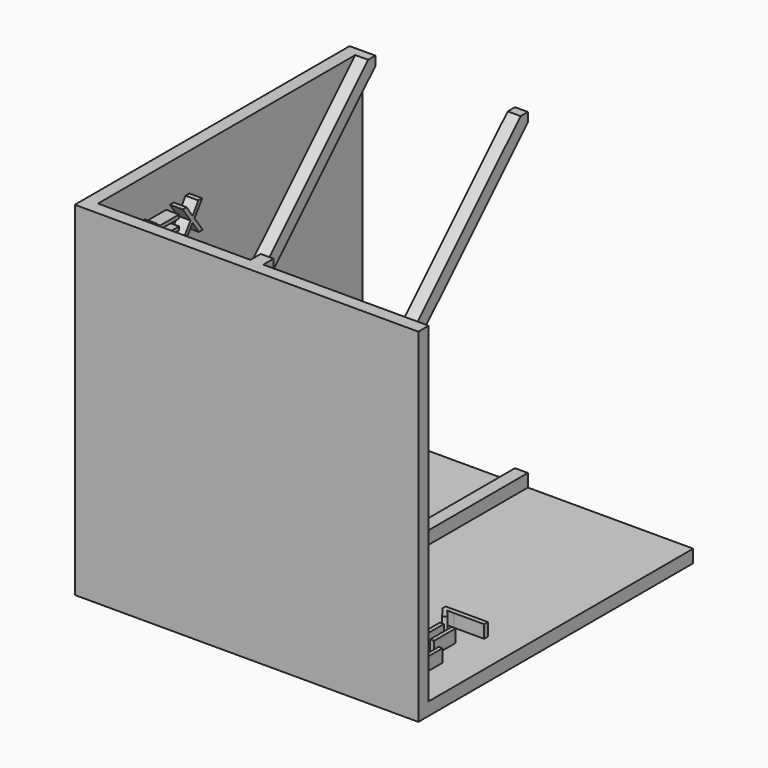
from build123d import *

# Parameters (mm, degrees)
F0_W          = 3.81
F0_H          = 203.2
F1_DEPTH      = 15.24
F0_W_2        = 97.79
F2_DEPTH      = 7.62
F3_W          = 97.79
F3_H          = 203.2
F4_DEPTH      = 7.62
F3_W_2        = 3.81
F5_DEPTH      = 15.24
F7_START      = 97.79
F7_DEPTH      = 7.62
F8_DEPTH      = 7.62
F9_DEPTH      = 15.24
F10_TEXT_SIZE = 30.8931965032
F11_DEPTH     = 7.62
F12_TEXT_SIZE = 34.9516233068
F13_DEPTH     = 7.62
F14_TEXT_SIZE = 34.9516233068
F15_DEPTH     = 7.62
F16_TEXT_SIZE = 14.9528583912
F17_DEPTH     = 7.62


# Not quite as in the source:
# - Text() gives the source's letters only with a copy of the font that has no kerning and outlines rounded to 1/6400 em; it was checked with that copy


with BuildPart() as f1:
    # F0 (on Top) → F1 (new body)
    with BuildSketch(Plane.XY):
        with Locations((99.695, 101.6)):
            Rectangle(F0_W, F0_H)
        with Locations((103.505, 101.6)):
            Rectangle(F0_W, F0_H)
    extrude(amount=F1_DEPTH)

    # F0 (on Top) → F2 (join)
    with BuildSketch(Plane.XY):
        with Locations((154.305, 101.6)):
            Rectangle(F0_W_2, F0_H)
        with Locations((48.895, 101.6)):
            Rectangle(F0_W_2, F0_H)
    extrude(amount=F2_DEPTH)

    # F3 (on Front) → F4 (join)
    with BuildSketch(Plane.XZ):
        with Locations((154.305, 101.6)):
            Rectangle(F3_W, F3_H)
        with Locations((48.895, 101.6)):
            Rectangle(F3_W, F3_H)
    extrude(amount=-F4_DEPTH)

    # F3 (on Front) → F5 (join)
    with BuildSketch(Plane.XZ):
        with Locations((103.505, 101.6)):
            Rectangle(F3_W_2, F3_H)
        with Locations((99.695, 101.6)):
            Rectangle(F3_W_2, F3_H)
    extrude(amount=-F5_DEPTH)

    # F6 (on Right) → F7 (join)
    with BuildSketch(Plane.YZ.offset(F7_START)):
        Polygon((0, 5.3881536726), (0, 0), (203.2, 203.2), (197.8118463274, 203.2), align=None)
        Polygon((203.2, 203.2), (0, 0), (5.3881536726, 0), (203.2, 197.8118463274), align=None)
    extrude(amount=F7_DEPTH)

    # F6 (on Right) → F8 (join)
    with BuildSketch(Plane.YZ):
        Polygon((0, 203.2), (0, 5.3881536726), (197.8118463274, 203.2), align=None)
        Polygon((203.2, 197.8118463274), (5.3881536726, 0), (203.2, 0), align=None)
    extrude(amount=F8_DEPTH)

    # F6 (on Right) → F9 (join)
    with BuildSketch(Plane.YZ):
        Polygon((0, 5.3881536726), (0, 0), (203.2, 203.2), (197.8118463274, 203.2), align=None)
        Polygon((203.2, 203.2), (0, 0), (5.3881536726, 0), (203.2, 197.8118463274), align=None)
    extrude(amount=F9_DEPTH)

    # F10 (on face) → F11 (join)
    with BuildSketch(Plane.YZ.offset(7.62)):
        with Locations((26.67, 164.4468985177)):
            Text('y=x', F10_TEXT_SIZE, font='Open Sans', text_align=(TextAlign.LEFT, TextAlign.BOTTOM))
    extrude(amount=F11_DEPTH)

    # F12 (on face) → F13 (join)
    with BuildSketch(Plane(origin=(0, 7.62, 0), x_dir=(-1, 0, 0), z_dir=(0, 1, 0))):
        with Locations((-187.452, 154.6668312191)):
            Text('z=1', F12_TEXT_SIZE, font='Open Sans', text_align=(TextAlign.LEFT, TextAlign.BOTTOM))
    extrude(amount=F13_DEPTH)

    # F14 (on face) → F15 (join)
    with BuildSketch(Plane.XY.offset(7.62)):
        with Locations(Location((184.15, 26.67), (0, 0, 90))):
            Text('z=1', F14_TEXT_SIZE, font='Open Sans', text_align=(TextAlign.LEFT, TextAlign.BOTTOM))
    extrude(amount=F15_DEPTH)

    # F18: F17 across face


with BuildPart() as f17:
    # F16 (on face) → F17 (new body)
    with BuildSketch(Plane.YZ):
        with Locations((222.25, 173.383936286)):
            Text('Cole Lawrence', F16_TEXT_SIZE, font='Open Sans', text_align=(TextAlign.LEFT, TextAlign.BOTTOM))
        with Locations((222.25, 153.0480488739)):
            Text('6/10/17', F16_TEXT_SIZE, font='Open Sans', text_align=(TextAlign.LEFT, TextAlign.BOTTOM))
    extrude(amount=-F17_DEPTH)


with BuildPart() as f1_1:
    add(f1.part)
    add(f17.part.mirror(Plane(origin=(53.9744968335, 203.2, 54.7799467398), x_dir=(-1, 0, 0), z_dir=(0, 1, 0))))


solid = f1_1.part
